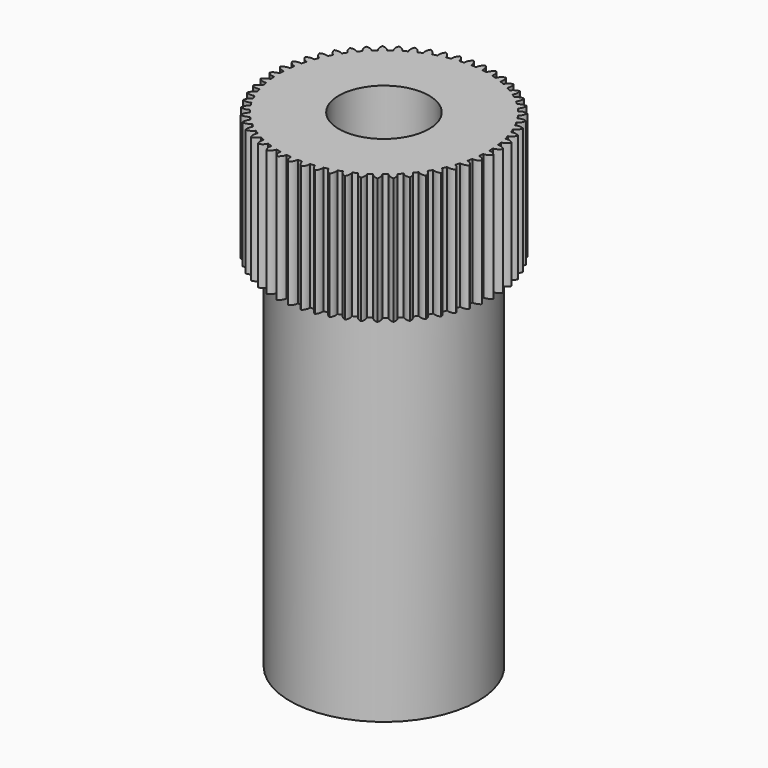
from build123d import *

# Parameters (mm, degrees)
F3_DEPTH        = 3.5
F3_COPIES_COUNT = 55


# Not quite as in the source:
# - a pattern or mirror of a feature is missing from the dataset's text; its kind, count and spacing are read off the source's solid


with BuildPart() as f1:
    # F0 (on Front) → F1 (revolve)
    with BuildSketch(Plane.XZ):
        Polygon((1.25, 13.5), (1.25, 0), (2.6, 0), (2.6, 10), (2.9, 10), (2.9, 13.5), align=None)
    revolve(axis=Axis((0, 0, 0.3942980568), (0, 0, 1)))

    # F2 (on face) → F3 (join, through all)
    with BuildSketch(Plane.XY.offset(13.5)):
        with BuildLine():
            ThreePointArc((-0.1, 2.8982753492), (0, 2.9), (0.1, 2.8982753492))
            ThreePointArc((0.1, 2.8982753492), (0.0736067977, 3.0100787481), (0, 3.0982753492))
            ThreePointArc((0, 3.0982753492), (-0.0736067977, 3.0100787481), (-0.1, 2.8982753492))
        make_face()
    f3 = extrude(amount=-F3_DEPTH)

    # F3_copies: F3 ×55 about axis
    f3_copies_axis = Axis((0, 0, 0), (0, 0, 1))
    for i in range(1, F3_COPIES_COUNT):
        add(f3.rotate(f3_copies_axis, i * 360 / F3_COPIES_COUNT))


solid = f1.part
